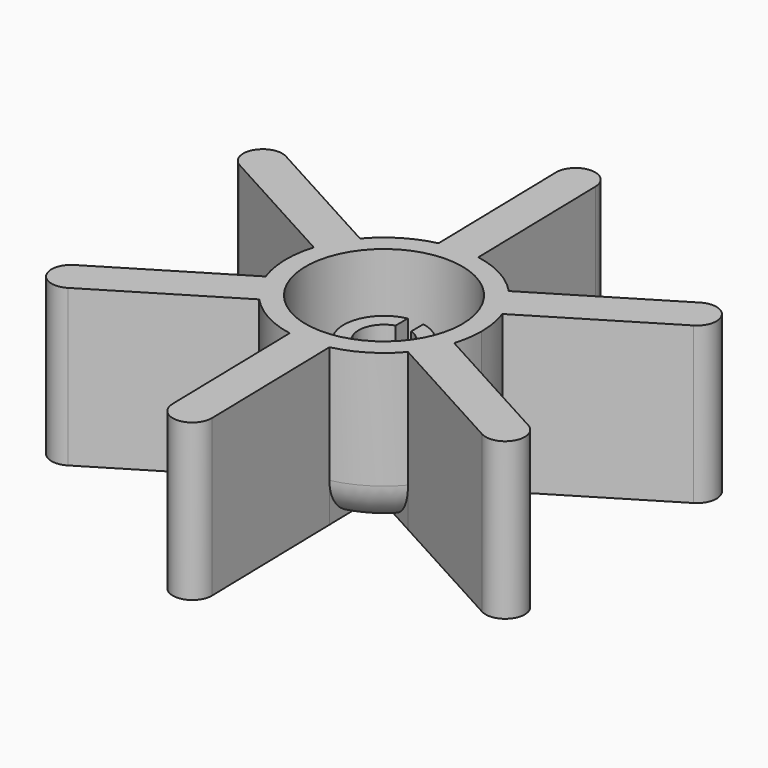
from build123d import *

# Parameters (mm, degrees)
F1_DEPTH     = 10
F2_DEPTH     = 5
F0_R         = 10
F3_DEPTH     = 15
F4_DEPTH     = 5
F6_T4_ANGLE  = 151.525388132
F6_T10_ANGLE = 151.525388132
F6_T16_ANGLE = 151.525388132
F6_T22_ANGLE = 151.525388132
F6_T28_ANGLE = 151.525388132
F6_T34_ANGLE = 151.525388132


# Not quite as in the source:
# - a fillet or chamfer that OpenCascade refuses, or shapes differently, is made with other operations: its cross-section is extruded or revolved along the edge and cut away or added
# - a feature of the source that left no trace in its solid (it failed there, or was rolled back) is left out


with BuildPart() as f1:
    # F0 (on Top) → F1 (new body)
    with BuildSketch(Plane.XY):
        with BuildLine():
            ThreePointArc((-3.1, -0.9759610648), (-2.8879484862, 1.4907224897), (-1, 3.0923292192))
            Line((-1, 3.0923292192), (-1, 5.0519798099))
            ThreePointArc((-1, 5.0519798099), (0, -5.15), (1, 5.0519798099))
            Line((1, 5.0519798099), (1, 3.0923292192))
            ThreePointArc((1, 3.0923292192), (2.8879484862, 1.4907224897), (3.1, -0.9759610648))
            ThreePointArc((3.1, -0.9759610648), (0, -3.25), (-3.1, -0.9759610648))
        make_face()
    extrude(amount=F1_DEPTH)

    # F0 (on Top) → F2 (join)
    with BuildSketch(Plane.XY):
        with BuildLine():
            Line((3.1, -0.9759610648), (-3.1, -0.9759610648))
            ThreePointArc((-3.1, -0.9759610648), (0, -3.25), (3.1, -0.9759610648))
        make_face()
    extrude(amount=F2_DEPTH)



with BuildPart() as f3:
    # F0 (on Top) → F3 (new body)
    with BuildSketch(Plane.XY):
        with BuildLine():
            ThreePointArc((11.940314229, -3.6984991703), (12.3592865462, -1.870303737), (12.5, 0))
            ThreePointArc((12.5, 0), (12.3154429017, 2.1400621802), (11.7672214184, 4.2169301738))
            ThreePointArc((11.7672214184, 4.2169301738), (10.6860892314, 6.4851751664), (9.1731513519, 8.4913658663))
            ThreePointArc((9.1731513519, 8.4913658663), (6.0118371583, 10.9593710578), (2.2316420527, 12.2991777672))
            ThreePointArc((2.2316420527, 12.2991777672), (-0.2732818264, 12.4970123247), (-2.7671628772, 12.1898650366))
            ThreePointArc((-2.7671628772, 12.1898650366), (-6.4851751664, 10.6860892314), (-9.5355793657, 8.0822475934))
            ThreePointArc((-9.5355793657, 8.0822475934), (-10.9593710578, 6.0118371583), (-11.940314229, 3.6984991703))
            ThreePointArc((-11.940314229, 3.6984991703), (-12.4970123247, -0.2732818264), (-11.7672214184, -4.2169301738))
            ThreePointArc((-11.7672214184, -4.2169301738), (-10.6860892314, -6.4851751664), (-9.1731513519, -8.4913658663))
            ThreePointArc((-9.1731513519, -8.4913658663), (-6.0118371583, -10.9593710578), (-2.2316420527, -12.2991777672))
            ThreePointArc((-2.2316420527, -12.2991777672), (0.2732818264, -12.4970123247), (2.7671628772, -12.1898650366))
            ThreePointArc((2.7671628772, -12.1898650366), (6.4851751664, -10.6860892314), (9.5355793657, -8.0822475934))
            ThreePointArc((9.5355793657, -8.0822475934), (10.9593710578, -6.0118371583), (11.940314229, -3.6984991703))
        make_face()
        Circle(F0_R, mode=Mode.SUBTRACT)
        with BuildLine():
            ThreePointArc((9.1731513519, 8.4913658663), (10.6860892314, 6.4851751664), (11.7672214184, 4.2169301738))
            Line((11.7672214184, 4.2169301738), (28.2476592825, 14.2185803615))
            ThreePointArc((28.2476592825, 14.2185803615), (29.3790077487, 15.7616992433), (29.0878420955, 17.652833241))
            ThreePointArc((29.0878420955, 17.652833241), (27.5447232138, 18.7841817072), (25.653589216, 18.4930160541))
            Line((25.653589216, 18.4930160541), (9.1731513519, 8.4913658663))
        make_face()
        with BuildLine():
            ThreePointArc((-2.7671628772, 12.1898650366), (-0.2732818264, 12.4970123247), (2.2316420527, 12.2991777672))
            Line((2.2316420527, 12.2991777672), (1.8101778425, 31.5724807169))
            ThreePointArc((1.8101778425, 31.5724807169), (1.0394719229, 33.32381667), (-0.7438809877, 34.0172268165))
            ThreePointArc((-0.7438809877, 34.0172268165), (-2.4952169409, 33.246520897), (-3.1886270874, 31.4631679863))
            Line((-3.1886270874, 31.4631679863), (-2.7671628772, 12.1898650366))
        make_face()
        with BuildLine():
            ThreePointArc((-11.940314229, 3.6984991703), (-10.9593710578, 6.0118371583), (-9.5355793657, 8.0822475934))
            Line((-9.5355793657, 8.0822475934), (-26.4374814401, 17.3539003554))
            ThreePointArc((-26.4374814401, 17.3539003554), (-28.3395358258, 17.5621174267), (-29.8317230833, 16.3643935755))
            ThreePointArc((-29.8317230833, 16.3643935755), (-30.0399401546, 14.4623391897), (-28.8422163034, 12.9701519323))
            Line((-28.8422163034, 12.9701519323), (-11.940314229, 3.6984991703))
        make_face()
        with BuildLine():
            Line((-25.653589216, -18.4930160541), (-9.1731513519, -8.4913658663))
            ThreePointArc((-9.1731513519, -8.4913658663), (-10.6860892314, -6.4851751664), (-11.7672214184, -4.2169301738))
            Line((-11.7672214184, -4.2169301738), (-28.2476592825, -14.2185803615))
            ThreePointArc((-28.2476592825, -14.2185803615), (-29.3790077487, -15.7616992433), (-29.0878420955, -17.652833241))
            ThreePointArc((-29.0878420955, -17.652833241), (-27.5447232138, -18.7841817072), (-25.653589216, -18.4930160541))
        make_face()
        with BuildLine():
            Line((3.1886270874, -31.4631679863), (2.7671628772, -12.1898650366))
            ThreePointArc((2.7671628772, -12.1898650366), (0.2732818264, -12.4970123247), (-2.2316420527, -12.2991777672))
            Line((-2.2316420527, -12.2991777672), (-1.8101778425, -31.5724807169))
            ThreePointArc((-1.8101778425, -31.5724807169), (-1.0394719229, -33.32381667), (0.7438809877, -34.0172268165))
            ThreePointArc((0.7438809877, -34.0172268165), (2.4952169409, -33.246520897), (3.1886270874, -31.4631679863))
        make_face()
        with BuildLine():
            Line((28.8422163034, -12.9701519323), (11.940314229, -3.6984991703))
            ThreePointArc((11.940314229, -3.6984991703), (10.9593710578, -6.0118371583), (9.5355793657, -8.0822475934))
            Line((9.5355793657, -8.0822475934), (26.4374814401, -17.3539003554))
            ThreePointArc((26.4374814401, -17.3539003554), (28.3395358258, -17.5621174267), (29.8317230833, -16.3643935755))
            ThreePointArc((29.8317230833, -16.3643935755), (30.0399401546, -14.4623391897), (28.8422163034, -12.9701519323))
        make_face()
    extrude(amount=F3_DEPTH)


with BuildPart() as f1_1:
    add(f1.part)

    add(f3.part)  # F4 merges F3
    # F0 (on Top) → F4 (join)
    with BuildSketch(Plane.XY):
        with BuildLine():
            ThreePointArc((11.940314229, -3.6984991703), (12.3592865462, -1.870303737), (12.5, 0))
            ThreePointArc((12.5, 0), (12.3154429017, 2.1400621802), (11.7672214184, 4.2169301738))
            ThreePointArc((11.7672214184, 4.2169301738), (10.6860892314, 6.4851751664), (9.1731513519, 8.4913658663))
            ThreePointArc((9.1731513519, 8.4913658663), (6.0118371583, 10.9593710578), (2.2316420527, 12.2991777672))
            ThreePointArc((2.2316420527, 12.2991777672), (-0.2732818264, 12.4970123247), (-2.7671628772, 12.1898650366))
            ThreePointArc((-2.7671628772, 12.1898650366), (-6.4851751664, 10.6860892314), (-9.5355793657, 8.0822475934))
            ThreePointArc((-9.5355793657, 8.0822475934), (-10.9593710578, 6.0118371583), (-11.940314229, 3.6984991703))
            ThreePointArc((-11.940314229, 3.6984991703), (-12.4970123247, -0.2732818264), (-11.7672214184, -4.2169301738))
            ThreePointArc((-11.7672214184, -4.2169301738), (-10.6860892314, -6.4851751664), (-9.1731513519, -8.4913658663))
            ThreePointArc((-9.1731513519, -8.4913658663), (-6.0118371583, -10.9593710578), (-2.2316420527, -12.2991777672))
            ThreePointArc((-2.2316420527, -12.2991777672), (0.2732818264, -12.4970123247), (2.7671628772, -12.1898650366))
            ThreePointArc((2.7671628772, -12.1898650366), (6.4851751664, -10.6860892314), (9.5355793657, -8.0822475934))
            ThreePointArc((9.5355793657, -8.0822475934), (10.9593710578, -6.0118371583), (11.940314229, -3.6984991703))
        make_face()
        Circle(F0_R, mode=Mode.SUBTRACT)
        with BuildLine():
            ThreePointArc((9.1731513519, 8.4913658663), (10.6860892314, 6.4851751664), (11.7672214184, 4.2169301738))
            Line((11.7672214184, 4.2169301738), (28.2476592825, 14.2185803615))
            ThreePointArc((28.2476592825, 14.2185803615), (29.3790077487, 15.7616992433), (29.0878420955, 17.652833241))
            ThreePointArc((29.0878420955, 17.652833241), (27.5447232138, 18.7841817072), (25.653589216, 18.4930160541))
            Line((25.653589216, 18.4930160541), (9.1731513519, 8.4913658663))
        make_face()
        with BuildLine():
            Line((28.8422163034, -12.9701519323), (11.940314229, -3.6984991703))
            ThreePointArc((11.940314229, -3.6984991703), (10.9593710578, -6.0118371583), (9.5355793657, -8.0822475934))
            Line((9.5355793657, -8.0822475934), (26.4374814401, -17.3539003554))
            ThreePointArc((26.4374814401, -17.3539003554), (28.3395358258, -17.5621174267), (29.8317230833, -16.3643935755))
            ThreePointArc((29.8317230833, -16.3643935755), (30.0399401546, -14.4623391897), (28.8422163034, -12.9701519323))
        make_face()
        with BuildLine():
            ThreePointArc((-2.7671628772, 12.1898650366), (-0.2732818264, 12.4970123247), (2.2316420527, 12.2991777672))
            Line((2.2316420527, 12.2991777672), (1.8101778425, 31.5724807169))
            ThreePointArc((1.8101778425, 31.5724807169), (1.0394719229, 33.32381667), (-0.7438809877, 34.0172268165))
            ThreePointArc((-0.7438809877, 34.0172268165), (-2.4952169409, 33.246520897), (-3.1886270874, 31.4631679863))
            Line((-3.1886270874, 31.4631679863), (-2.7671628772, 12.1898650366))
        make_face()
        with BuildLine():
            Line((3.1886270874, -31.4631679863), (2.7671628772, -12.1898650366))
            ThreePointArc((2.7671628772, -12.1898650366), (0.2732818264, -12.4970123247), (-2.2316420527, -12.2991777672))
            Line((-2.2316420527, -12.2991777672), (-1.8101778425, -31.5724807169))
            ThreePointArc((-1.8101778425, -31.5724807169), (-1.0394719229, -33.32381667), (0.7438809877, -34.0172268165))
            ThreePointArc((0.7438809877, -34.0172268165), (2.4952169409, -33.246520897), (3.1886270874, -31.4631679863))
        make_face()
        with BuildLine():
            ThreePointArc((-11.940314229, 3.6984991703), (-10.9593710578, 6.0118371583), (-9.5355793657, 8.0822475934))
            Line((-9.5355793657, 8.0822475934), (-26.4374814401, 17.3539003554))
            ThreePointArc((-26.4374814401, 17.3539003554), (-28.3395358258, 17.5621174267), (-29.8317230833, 16.3643935755))
            ThreePointArc((-29.8317230833, 16.3643935755), (-30.0399401546, 14.4623391897), (-28.8422163034, 12.9701519323))
            Line((-28.8422163034, 12.9701519323), (-11.940314229, 3.6984991703))
        make_face()
        with BuildLine():
            Line((-25.653589216, -18.4930160541), (-9.1731513519, -8.4913658663))
            ThreePointArc((-9.1731513519, -8.4913658663), (-10.6860892314, -6.4851751664), (-11.7672214184, -4.2169301738))
            Line((-11.7672214184, -4.2169301738), (-28.2476592825, -14.2185803615))
            ThreePointArc((-28.2476592825, -14.2185803615), (-29.3790077487, -15.7616992433), (-29.0878420955, -17.652833241))
            ThreePointArc((-29.0878420955, -17.652833241), (-27.5447232138, -18.7841817072), (-25.653589216, -18.4930160541))
        make_face()
        Circle(F0_R)
        with BuildLine():
            Line((-1, 5.0519798099), (-1, 3.0923292192))
            ThreePointArc((-1, 3.0923292192), (-2.8879484862, 1.4907224897), (-3.1, -0.9759610648))
            Line((-3.1, -0.9759610648), (3.1, -0.9759610648))
            ThreePointArc((3.1, -0.9759610648), (2.8879484862, 1.4907224897), (1, 3.0923292192))
            Line((1, 3.0923292192), (1, 5.0519798099))
            ThreePointArc((1, 5.0519798099), (0, -5.15), (-1, 5.0519798099))
        make_face(mode=Mode.SUBTRACT)
        with BuildLine():
            Line((3.1, -0.9759610648), (-3.1, -0.9759610648))
            ThreePointArc((-3.1, -0.9759610648), (0, -3.25), (3.1, -0.9759610648))
        make_face()
        with BuildLine():
            ThreePointArc((-3.1, -0.9759610648), (-2.8879484862, 1.4907224897), (-1, 3.0923292192))
            Line((-1, 3.0923292192), (-1, 5.0519798099))
            ThreePointArc((-1, 5.0519798099), (0, -5.15), (1, 5.0519798099))
            Line((1, 5.0519798099), (1, 3.0923292192))
            ThreePointArc((1, 3.0923292192), (2.8879484862, 1.4907224897), (3.1, -0.9759610648))
            ThreePointArc((3.1, -0.9759610648), (0, -3.25), (-3.1, -0.9759610648))
        make_face()
    extrude(amount=-F4_DEPTH)

    # F6: fillet of radius 5 on 6 edges, made by hand


with BuildPart() as f6_tool2:
    # F6_s3 → F6_t4 (revolve)
    with BuildSketch(Plane(origin=(0, 0, 0), x_dir=(0, 0, 1), z_dir=(0.9636769063, 0.2670708152, 0))):
        with BuildLine():
            ThreePointArc((-5, -7.5), (-3.5355339059, -11.0355339059), (0, -12.5))
            Line((0, -12.5), (0, -12.6))
            Line((0, -12.6), (-5.1, -12.6))
            Line((-5.1, -12.6), (-5.1, -7.5))
            Line((-5.1, -7.5), (-5, -7.5))
        make_face()
    revolve(axis=Axis((0, 0, -5), (0, 0, 1)), revolution_arc=F6_T4_ANGLE)

    split(bisect_by=Plane(origin=(-1.2023674317, -2.1918742116, 0), x_dir=(0, 0, 1), z_dir=(-0.4809469727, -0.8767496846, 0)), keep=Keep.TOP)

    split(bisect_by=Plane(origin=(-1.2970350333, 2.1372178463, 0), x_dir=(0, 0, 1), z_dir=(-0.5188140133, 0.8548871385, 0)), keep=Keep.TOP)


with BuildPart() as f1_2:
    add(f1_1.part)

    # F6_t1: cut F6_tool2
    add(f6_tool2.part, mode=Mode.SUBTRACT)


with BuildPart() as f6_tool8:
    # F6_s9 → F6_t10 (revolve)
    with BuildSketch(Plane(origin=(0, 0, 0), x_dir=(0, 0, 1), z_dir=(-0.2505483426, -0.9681040895, 0))):
        with BuildLine():
            ThreePointArc((0, -12.5), (-3.5355339059, -11.0355339059), (-5, -7.5))
            Line((-5, -7.5), (-5.1, -7.5))
            Line((-5.1, -7.5), (-5.1, -12.6))
            Line((-5.1, -12.6), (0, -12.6))
            Line((0, -12.6), (0, -12.5))
        make_face()
    revolve(axis=Axis((0, 0, -5), (0, 0, 1)), revolution_arc=F6_T10_ANGLE)

    split(bisect_by=Plane(origin=(-1.2970350333, 2.1372178463, 0), x_dir=(0, 0, 1), z_dir=(-0.5188140133, 0.8548871385, 0)), keep=Keep.TOP)

    split(bisect_by=Plane(origin=(2.4994024649, 0.0546563653, 0), x_dir=(0, 0, 1), z_dir=(0.999760986, 0.0218625461, 0)), keep=Keep.TOP)


with BuildPart() as f1_3:
    add(f1_2.part)

    # F6_t7: cut F6_tool8
    add(f6_tool8.part, mode=Mode.SUBTRACT)


with BuildPart() as f6_tool14:
    # F6_s15 → F6_t16 (revolve)
    with BuildSketch(Plane(origin=(0, 0, 0), x_dir=(0, 0, 1), z_dir=(0.7131285637, -0.7010332743, 0))):
        with BuildLine():
            ThreePointArc((-5, -7.5), (-3.5355339059, -11.0355339059), (0, -12.5))
            Line((0, -12.5), (0, -12.6))
            Line((0, -12.6), (-5.1, -12.6))
            Line((-5.1, -12.6), (-5.1, -7.5))
            Line((-5.1, -7.5), (-5, -7.5))
        make_face()
    revolve(axis=Axis((0, 0, -5), (0, 0, 1)), revolution_arc=F6_T16_ANGLE)

    split(bisect_by=Plane(origin=(-2.4994024649, -0.0546563653, 0), x_dir=(0, 0, 1), z_dir=(-0.999760986, -0.0218625461, 0)), keep=Keep.TOP)

    split(bisect_by=Plane(origin=(1.2023674317, 2.1918742116, 0), x_dir=(0, 0, 1), z_dir=(0.4809469727, 0.8767496846, 0)), keep=Keep.TOP)


with BuildPart() as f1_4:
    add(f1_3.part)

    # F6_t13: cut F6_tool14
    add(f6_tool14.part, mode=Mode.SUBTRACT)


with BuildPart() as f6_tool20:
    # F6_s21 → F6_t22 (revolve)
    with BuildSketch(Plane(origin=(0, 0, 0), x_dir=(0, 0, 1), z_dir=(0.2505483426, 0.9681040895, 0))):
        with BuildLine():
            ThreePointArc((-5, -7.5), (-3.5355339059, -11.0355339059), (0, -12.5))
            Line((0, -12.5), (0, -12.6))
            Line((0, -12.6), (-5.1, -12.6))
            Line((-5.1, -12.6), (-5.1, -7.5))
            Line((-5.1, -7.5), (-5, -7.5))
        make_face()
    revolve(axis=Axis((0, 0, -5), (0, 0, 1)), revolution_arc=F6_T22_ANGLE)

    split(bisect_by=Plane(origin=(1.2970350333, -2.1372178463, 0), x_dir=(0, 0, 1), z_dir=(0.5188140133, -0.8548871385, 0)), keep=Keep.TOP)

    split(bisect_by=Plane(origin=(-2.4994024649, -0.0546563653, 0), x_dir=(0, 0, 1), z_dir=(-0.999760986, -0.0218625461, 0)), keep=Keep.TOP)


with BuildPart() as f1_5:
    add(f1_4.part)

    # F6_t19: cut F6_tool20
    add(f6_tool20.part, mode=Mode.SUBTRACT)


with BuildPart() as f6_tool26:
    # F6_s27 → F6_t28 (revolve)
    with BuildSketch(Plane(origin=(0, 0, 0), x_dir=(0, 0, 1), z_dir=(-0.7131285637, 0.7010332743, 0))):
        with BuildLine():
            ThreePointArc((-5, -7.5), (-3.5355339059, -11.0355339059), (0, -12.5))
            Line((0, -12.5), (0, -12.6))
            Line((0, -12.6), (-5.1, -12.6))
            Line((-5.1, -12.6), (-5.1, -7.5))
            Line((-5.1, -7.5), (-5, -7.5))
        make_face()
    revolve(axis=Axis((0, 0, -5), (0, 0, 1)), revolution_arc=F6_T28_ANGLE)

    split(bisect_by=Plane(origin=(2.4994024649, 0.0546563653, 0), x_dir=(0, 0, 1), z_dir=(0.999760986, 0.0218625461, 0)), keep=Keep.TOP)

    split(bisect_by=Plane(origin=(-1.2023674317, -2.1918742116, 0), x_dir=(0, 0, 1), z_dir=(-0.4809469727, -0.8767496846, 0)), keep=Keep.TOP)


with BuildPart() as f1_6:
    add(f1_5.part)

    # F6_t25: cut F6_tool26
    add(f6_tool26.part, mode=Mode.SUBTRACT)


with BuildPart() as f6_tool32:
    # F6_s33 → F6_t34 (revolve)
    with BuildSketch(Plane(origin=(0, 0, 0), x_dir=(0, 0, 1), z_dir=(-0.9636769063, -0.2670708152, 0))):
        with BuildLine():
            ThreePointArc((-5, -7.5), (-3.5355339059, -11.0355339059), (0, -12.5))
            Line((0, -12.5), (0, -12.6))
            Line((0, -12.6), (-5.1, -12.6))
            Line((-5.1, -12.6), (-5.1, -7.5))
            Line((-5.1, -7.5), (-5, -7.5))
        make_face()
    revolve(axis=Axis((0, 0, -5), (0, 0, 1)), revolution_arc=F6_T34_ANGLE)

    split(bisect_by=Plane(origin=(1.2023674317, 2.1918742116, 0), x_dir=(0, 0, 1), z_dir=(0.4809469727, 0.8767496846, 0)), keep=Keep.TOP)

    split(bisect_by=Plane(origin=(1.2970350333, -2.1372178463, 0), x_dir=(0, 0, 1), z_dir=(0.5188140133, -0.8548871385, 0)), keep=Keep.TOP)


with BuildPart() as f1_7:
    add(f1_6.part)

    # F6_t31: cut F6_tool32
    add(f6_tool32.part, mode=Mode.SUBTRACT)


solid = f1_7.part
